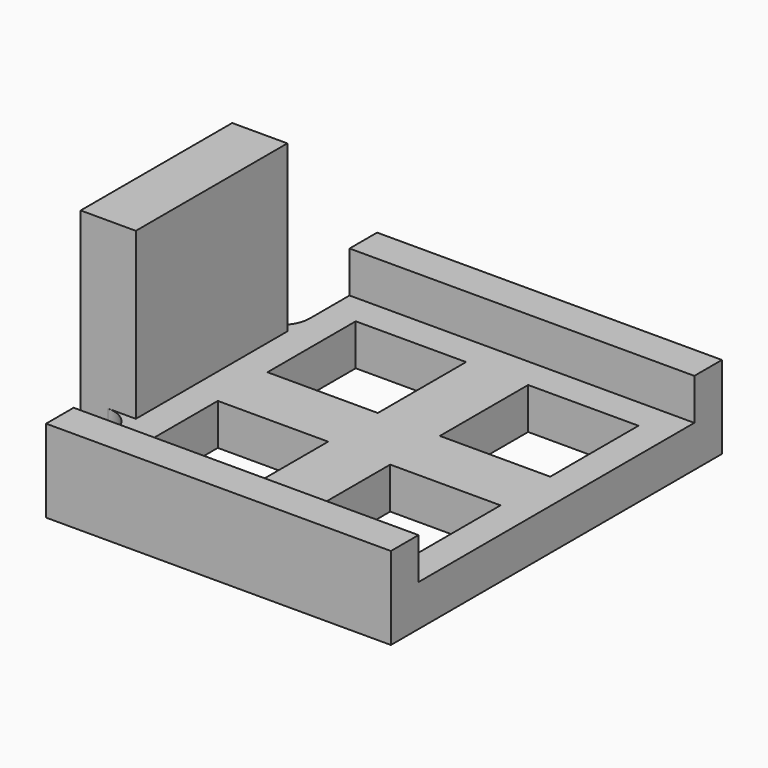
from build123d import *

# Parameters (mm, degrees)
F0_W     = 25
F0_H     = 30
F1_DEPTH = 3
F2_W     = 25
F2_H     = 2.5
F3_DEPTH = 3
F4_W     = 4
F4_H     = 13.7322908992
F5_DEPTH = 15
F6_R     = 2
F7_W     = 8
F7_H     = 8
F8_DEPTH = 3


with BuildPart() as f1:
    # F0 (on Top) → F1 (new body)
    with BuildSketch(Plane.XY):
        Rectangle(F0_W, F0_H)
    extrude(amount=F1_DEPTH)

    # F2 (on face) → F3 (join)
    with BuildSketch(Plane.XY.offset(3)):
        with Locations((0, 13.75)):
            Rectangle(F2_W, F2_H)
        with Locations((0, -13.75)):
            Rectangle(F2_W, F2_H)
    extrude(amount=F3_DEPTH)

    # F4 (on Top) → F5 (join)
    with BuildSketch(Plane.XY):
        with Locations((-14.5, 0)):
            Rectangle(F4_W, F4_H)
    extrude(amount=F5_DEPTH)

    # F6
    f6_edges = [f1.edges().sort_by_distance(p)[0] for p in [
        (-12.5, -6.866145, 1.5),
        (-12.5, 6.866145, 1.5),
    ]]
    fillet(f6_edges, radius=F6_R)

    # F7 (on face) → F8 (cut)
    with BuildSketch(Plane.XY.offset(3)):
        with Locations((-6.25, 6.25)):
            Rectangle(F7_W, F7_H)
        with Locations((6.25, 6.25)):
            Rectangle(F7_W, F7_H)
        with Locations((-6.25, -6.25)):
            Rectangle(F7_W, F7_H)
        with Locations((6.25, -6.25)):
            Rectangle(F7_W, F7_H)
    extrude(amount=-F8_DEPTH, mode=Mode.SUBTRACT)


solid = f1.part
